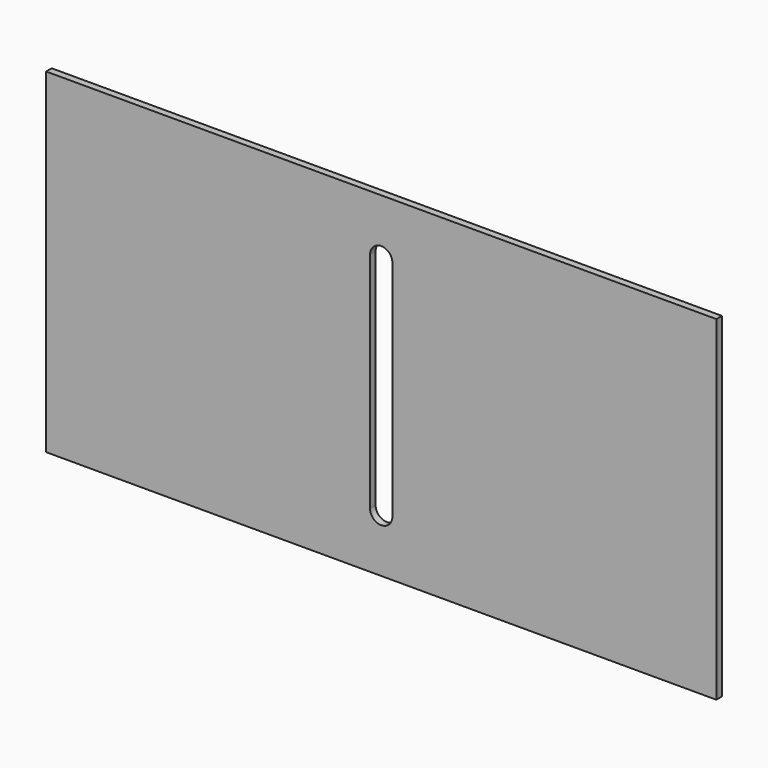
from build123d import *

# Parameters (mm, degrees)
F0_W     = 152.4
F0_H     = 76.2
F1_DEPTH = 1.5875
F2_W     = 5.08
F2_H     = 50.8
F3_DEPTH = 25.4
F5_DEPTH = 25.4


# Not quite as in the source:
# - a length typed as a fraction of an inch, garbled in the dataset ("3 / 203.2 mm" for 3/8 in), is restored


with BuildPart() as f1:
    # F0 (on Front) → F1 (new body)
    with BuildSketch(Plane.XZ):
        Rectangle(F0_W, F0_H)
    extrude(amount=F1_DEPTH)

    # F2 (on face) → F3 (cut)
    with BuildSketch(Plane.XZ.offset(1.5875)):
        Rectangle(F2_W, F2_H)
    extrude(amount=-F3_DEPTH, mode=Mode.SUBTRACT)

    # F4 (on face) → F5 (cut)
    with BuildSketch(Plane.XZ.offset(1.5875)):
        with BuildLine():
            Line((2.54, -25.4), (-2.54, -25.4))
            ThreePointArc((-2.54, -25.4), (0, -27.94), (2.54, -25.4))
        make_face()
        with BuildLine():
            ThreePointArc((2.54, 25.4), (0, 27.94), (-2.54, 25.4))
            Line((-2.54, 25.4), (2.54, 25.4))
        make_face()
    extrude(amount=-F5_DEPTH, mode=Mode.SUBTRACT)


solid = f1.part
